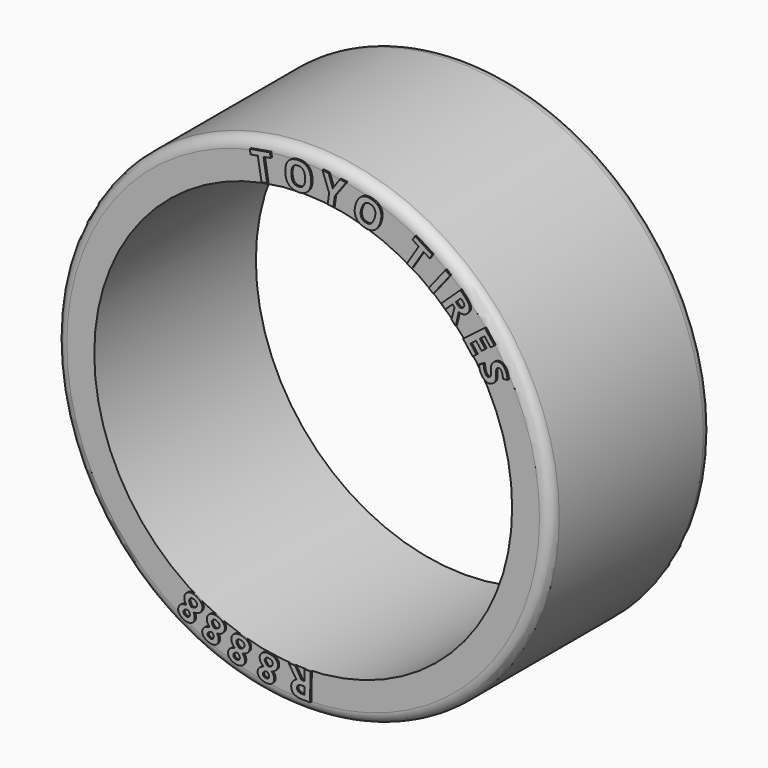
from build123d import *

# Parameters (mm, degrees)
F0_R           = 373.1264411569
F0_R_2         = 315.2396742934
F1_DEPTH       = 304.8
F2_R           = 16.51
F3_TEXT_SIZE   = 57.095728776
F3_TEXT_SIZE_2 = 57.6048289746
F3_TEXT_SIZE_3 = 57.8877756983
F3_TEXT_SIZE_4 = 57.3944497452
F3_TEXT_SIZE_5 = 56.8555013162
F3_TEXT_SIZE_6 = 57.3883969835
F3_TEXT_SIZE_7 = 55.5703684498
F3_TEXT_SIZE_8 = 57.6995797867
F3_TEXT_SIZE_9 = 55.1395719974
F4_DEPTH       = 2.54
F5_TEXT_SIZE   = 58.052753443
F5_TEXT_SIZE_2 = 55.0869264889
F5_TEXT_SIZE_3 = 56.4250662337
F5_TEXT_SIZE_4 = 55.5117961959
F5_TEXT_SIZE_5 = 56.633081554
F6_DEPTH       = 2.54


# Not quite as in the source:
# - Text() gives the source's letters only with a copy of the font that has no kerning and outlines rounded to 1/6400 em; it was checked with that copy


with BuildPart() as f1:
    # F0 (on Front) → F1 (new body)
    with BuildSketch(Plane.XZ):
        Circle(F0_R)
        Circle(F0_R_2, mode=Mode.SUBTRACT)
    extrude(amount=F1_DEPTH)

    # F2
    f2_edges = [f1.edges().sort_by_distance(p)[0] for p in [
        (-373.126441, -304.8, 0),
        (-373.126441, 0, 0),
    ]]
    fillet(f2_edges, radius=F2_R)


with BuildPart() as f4:
    # F3 (on face) → F4 (new body)
    with BuildSketch(Plane.XZ.offset(304.8)):
        with Locations(Location((-72.8991425359, 309.4273025793), (0, 0, 9.5456353042))):
            Text('T', F3_TEXT_SIZE, font='Open Sans', font_style=FontStyle.BOLD, text_align=(TextAlign.LEFT, TextAlign.BOTTOM))
        with Locations(Location((-28.0886535696, 316.3491789026), (0, 0, 0.891898384))):
            Text('O', F3_TEXT_SIZE_2, font='Open Sans', font_style=FontStyle.BOLD, text_align=(TextAlign.LEFT, TextAlign.BOTTOM))
        with Locations(Location((25.3867671889, 316.3227899068), (0, 0, -7.9178371344))):
            Text('Y', F3_TEXT_SIZE_3, font='Open Sans', font_style=FontStyle.BOLD, text_align=(TextAlign.LEFT, TextAlign.BOTTOM))
        with Locations(Location((71.8210155273, 309.4511011791), (0, 0, -17.5647505691))):
            Text('O', F3_TEXT_SIZE_4, font='Open Sans', font_style=FontStyle.BOLD, text_align=(TextAlign.LEFT, TextAlign.BOTTOM))
        with Locations(Location((148.2660666328, 281.1140443836), (0, 0, -32.1017345598))):
            Text('T', F3_TEXT_SIZE_5, font='Open Sans', font_style=FontStyle.BOLD, text_align=(TextAlign.LEFT, TextAlign.BOTTOM))
        with Locations(Location((187.2956757941, 255.9596347369), (0, 0, -38.3031562408))):
            Text('I', F3_TEXT_SIZE_6, font='Open Sans', font_style=FontStyle.BOLD, text_align=(TextAlign.LEFT, TextAlign.BOTTOM))
        with Locations(Location((206.9989520206, 242.0962378793), (0, 0, -46.6736840031))):
            Text('R', F3_TEXT_SIZE_7, font='Open Sans', font_style=FontStyle.BOLD, text_align=(TextAlign.LEFT, TextAlign.BOTTOM))
        with Locations(Location((240.1841681113, 206.2459202021), (0, 0, -52.4318726357))):
            Text('E', F3_TEXT_SIZE_8, font='Open Sans', font_style=FontStyle.BOLD, text_align=(TextAlign.LEFT, TextAlign.BOTTOM))
        with Locations(Location((264.5708518969, 177.0852866737), (0, 0, -62.8433030401))):
            Text('S', F3_TEXT_SIZE_9, font='Open Sans', font_style=FontStyle.BOLD, text_align=(TextAlign.LEFT, TextAlign.BOTTOM))
    extrude(amount=F4_DEPTH)


with BuildPart() as f6:
    # F5 (on face) → F6 (new body)
    with BuildSketch(Plane.XZ.offset(304.8)):
        with Locations(Location((18.2990456396, -314.708114254), (0, 0, 179.0112085629))):
            Text('R', F5_TEXT_SIZE, font='Open Sans', font_style=FontStyle.BOLD, text_align=(TextAlign.LEFT, TextAlign.BOTTOM))
        with Locations(Location((-32.3987175124, -315.5098880721), (0, 0, 167.8050038142))):
            Text('8', F5_TEXT_SIZE_2, font='Open Sans', font_style=FontStyle.BOLD, text_align=(TextAlign.LEFT, TextAlign.BOTTOM))
        with Locations(Location((-74.1302878084, -306.6307482634), (0, 0, 162.9483445217))):
            Text('8', F5_TEXT_SIZE_3, font='Open Sans', font_style=FontStyle.BOLD, text_align=(TextAlign.LEFT, TextAlign.BOTTOM))
        with Locations(Location((-111.2839773566, -294.6236487237), (0, 0, 156.7873131189))):
            Text('8', F5_TEXT_SIZE_4, font='Open Sans', font_style=FontStyle.BOLD, text_align=(TextAlign.LEFT, TextAlign.BOTTOM))
        with Locations(Location((-144.6075752436, -279.8548485265), (0, 0, 149.9675135106))):
            Text('8', F5_TEXT_SIZE_5, font='Open Sans', font_style=FontStyle.BOLD, text_align=(TextAlign.LEFT, TextAlign.BOTTOM))
    extrude(amount=F6_DEPTH)


solid = Compound([f1.part, f4.part, f6.part])
